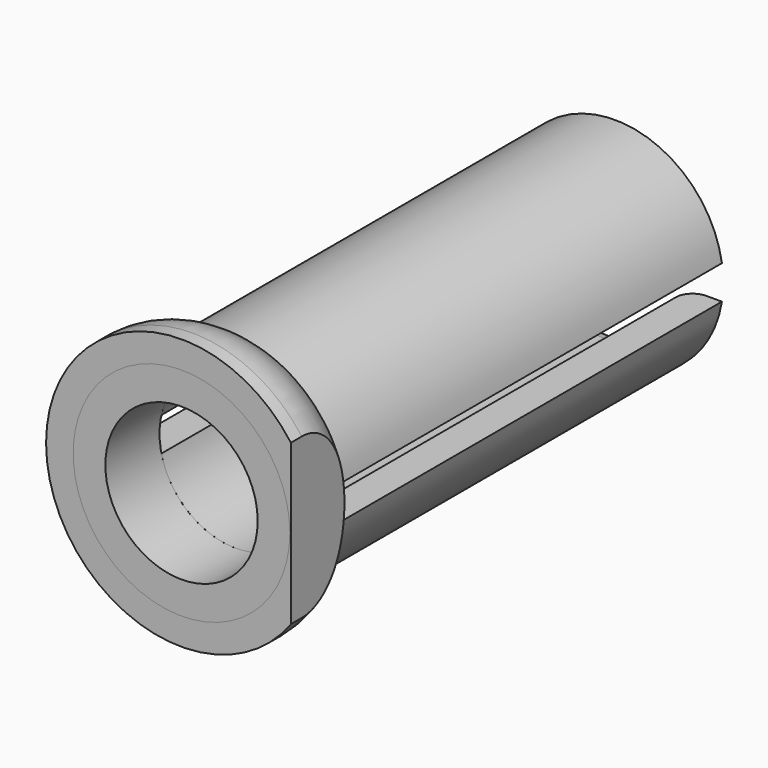
from build123d import *

# Parameters (mm, degrees)
F0_R      = 3.2
F0_R_2    = 2.25
F1_DEPTH  = 7
F2_R      = 0.5
F3_R      = 4
F3_R_2    = 3.2
F4_DEPTH  = 2
F6_DEPTH  = 2
F8_DEPTH  = 14
F10_DEPTH = 25


# Not quite as in the source:
# - a fillet or chamfer that OpenCascade refuses, or shapes differently, is made with other operations: its cross-section is extruded or revolved along the edge and cut away or added


with BuildPart() as f1:
    # F0 (on Front) → F1 (new body, symmetric)
    with BuildSketch(Plane.XZ):
        Circle(F0_R)
        Circle(F0_R_2, mode=Mode.SUBTRACT)
    extrude(amount=F1_DEPTH, both=True)

    # F2
    f2_edges = [f1.edges().sort_by_distance(p)[0] for p in [
        (-2.25, 7, 0),
    ]]
    fillet(f2_edges, radius=F2_R)

    # F3 (on face) → F4 (join)
    with BuildSketch(Plane.XZ.offset(7)):
        Circle(F3_R)
        Circle(F3_R_2, mode=Mode.SUBTRACT)
    extrude(amount=F4_DEPTH)

    # F5: fillet of radius 2 on 1 edges, made by hand

    # F5_s1 → F5_t2 (revolve, cut)
    with BuildSketch(Plane.XY):
        with BuildLine():
            ThreePointArc((4, -8.6), (3.788854382, -7.705572809), (3.2, -7))
            Line((3.2, -7), (4, -7))
            Line((4, -7), (4, -8.6))
        make_face()
    revolve(axis=Axis((0, -7, 0), (0, -1, 0)), mode=Mode.SUBTRACT)


with BuildPart() as f6:
    # F6 (new): a face of the model
    f6_faces = [f1.part.faces().sort_by_distance(p)[0] for p in [
        (-3.109490332, -7, 0),
    ]]
    extrude(f6_faces, amount=F6_DEPTH)


with BuildPart() as f1_1:
    add(f1.part)

    # F7 (on face) → F8 (cut)
    with BuildSketch(Plane(origin=(0, 7, 0), x_dir=(-1, 0, 0), z_dir=(0, 1, 0))):
        with BuildLine():
            Line((3.6153841381, -0.5), (3.6153841381, 0.5))
            Line((3.6153841381, 0.5), (3.1606961259, 0.5))
            ThreePointArc((3.1606961259, 0.5), (3.1901588991, 0.2507712077), (3.2, 0))
            ThreePointArc((3.2, 0), (3.1901588991, -0.2507712077), (3.1606961259, -0.5))
            Line((3.1606961259, -0.5), (3.6153841381, -0.5))
        make_face()
        with BuildLine():
            ThreePointArc((3.2, 0), (3.1901588991, 0.2507712077), (3.1606961259, 0.5))
            Line((3.1606961259, 0.5), (2.7041634566, 0.5))
            ThreePointArc((2.7041634566, 0.5), (2.7385168893, 0.2510482965), (2.75, 0))
            ThreePointArc((2.75, 0), (2.7385168893, -0.2510482965), (2.7041634566, -0.5))
            Line((2.7041634566, -0.5), (3.1606961259, -0.5))
            ThreePointArc((3.1606961259, -0.5), (3.1901588991, -0.2507712077), (3.2, 0))
        make_face()
        with BuildLine():
            ThreePointArc((2.75, 0), (2.7385168893, 0.2510482965), (2.7041634566, 0.5))
            Line((2.7041634566, 0.5), (-2.7041634566, 0.5))
            ThreePointArc((-2.7041634566, 0.5), (-2.75, 0), (-2.7041634566, -0.5))
            Line((-2.7041634566, -0.5), (2.7041634566, -0.5))
            ThreePointArc((2.7041634566, -0.5), (2.7385168893, -0.2510482965), (2.75, 0))
        make_face()
        with BuildLine():
            ThreePointArc((-3.1606961259, -0.5), (-3.2, 0), (-3.1606961259, 0.5))
            Line((-3.1606961259, 0.5), (-3.6153841381, 0.5))
            Line((-3.6153841381, 0.5), (-3.6153841381, -0.5))
            Line((-3.6153841381, -0.5), (-3.1606961259, -0.5))
        make_face()
        with BuildLine():
            Line((-2.7041634566, 0.5), (-3.1606961259, 0.5))
            ThreePointArc((-3.1606961259, 0.5), (-3.2, 0), (-3.1606961259, -0.5))
            Line((-3.1606961259, -0.5), (-2.7041634566, -0.5))
            ThreePointArc((-2.7041634566, -0.5), (-2.75, 0), (-2.7041634566, 0.5))
        make_face()
    extrude(amount=-F8_DEPTH, mode=Mode.SUBTRACT)

    # F9 (on face) → F10 (cut)
    with BuildSketch(Plane.XZ.offset(9)):
        with BuildLine():
            Line((3.2306045759, -2.3586424218), (3.2306045759, -4.3381056748))
            Line((3.2306045759, -4.3381056748), (4.7693954241, -4.3381056748))
            Line((4.7693954241, -4.3381056748), (4.7693954241, 4.3381056748))
            Line((4.7693954241, 4.3381056748), (3.2306045759, 4.3381056748))
            Line((3.2306045759, 4.3381056748), (3.2306045759, 2.3586424218))
            ThreePointArc((3.2306045759, 2.3586424218), (3.8027896539, 1.2404800878), (4, 0))
            ThreePointArc((4, 0), (3.8027896539, -1.2404800878), (3.2306045759, -2.3586424218))
        make_face()
        with BuildLine():
            Line((3.2306045759, 2.3586424218), (3.2306045759, -2.3586424218))
            ThreePointArc((3.2306045759, -2.3586424218), (3.8027896539, -1.2404800878), (4, 0))
            ThreePointArc((4, 0), (3.8027896539, 1.2404800878), (3.2306045759, 2.3586424218))
        make_face()
    extrude(amount=-F10_DEPTH, mode=Mode.SUBTRACT)


solid = Compound([f6.part, f1_1.part])
